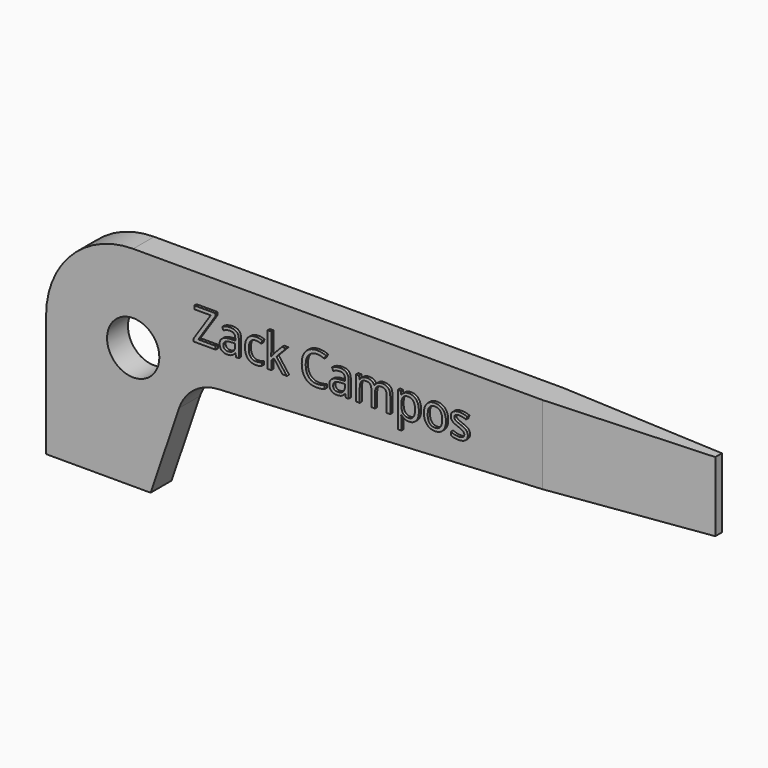
from build123d import *

# Parameters (mm, degrees)
F1_DEPTH     = 2.38125
F2_R         = 2.38125
F3_DEPTH     = 2.38225
F5_DEPTH     = 25.4
F6_TEXT_SIZE = 4.0851406026
F7_DEPTH     = 0.254


# Not quite as in the source:
# - Text() gives the source's letters only with a copy of the font that has no kerning and outlines rounded to 1/6400 em; it was checked with that copy


with BuildPart() as f1:
    # F0 (on Front) → F1 (new body)
    with BuildSketch(Plane.XZ):
        with BuildLine():
            Line((60.325, 19.05), (7.9375, 19.05))
            ThreePointArc((7.9375, 19.05), (2.3248399243, 16.7251600757), (0, 11.1125))
            Line((0, 11.1125), (0, 0))
            Line((0, 0), (9.525, 0))
            Line((9.525, 0), (12.1173647876, 7.6271664624))
            ThreePointArc((12.1173647876, 7.6271664624), (13.4786145605, 9.5135918491), (15.6631963617, 10.3130942181))
            Line((15.6631963617, 10.3130942181), (60.325, 12.7))
            Line((60.325, 12.7), (60.325, 19.05))
        make_face()
    extrude(amount=F1_DEPTH)

    # F2 (on face) → F3 (cut, through all)
    with BuildSketch(Plane.XZ.offset(2.38125)):
        with Locations((7.9375, 11.1125)):
            Circle(F2_R)
    extrude(amount=-F3_DEPTH, mode=Mode.SUBTRACT)

    # F4 (on face) → F5 (cut)
    with BuildSketch(Plane.XY.offset(19.05)):
        Polygon((60.325, -2.38125), (60.325, -1.56845), (45.24375, -2.38125), align=None)
        Polygon((45.24375, 0), (60.325, -0.8128), (60.325, 0), align=None)
    extrude(amount=-F5_DEPTH, mode=Mode.SUBTRACT)

    # F6 (on face) → F7 (join)
    with BuildSketch(Plane.XZ.offset(2.38125)):
        with Locations((13.49375, 13.5686987661)):
            Text('Zack Campos', F6_TEXT_SIZE, font='Open Sans', text_align=(TextAlign.LEFT, TextAlign.BOTTOM))
    extrude(amount=F7_DEPTH)


solid = f1.part
